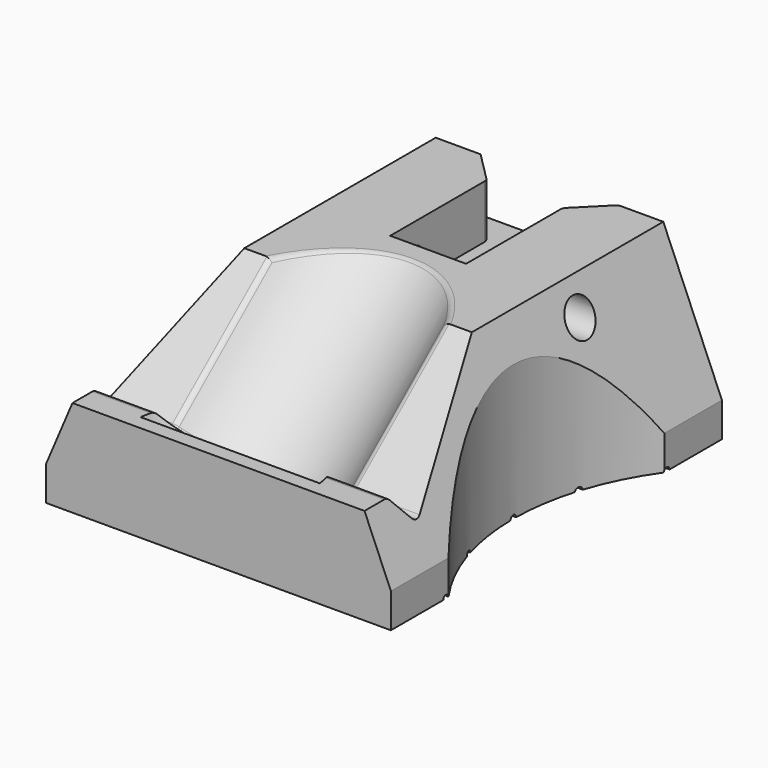
from build123d import *

# Parameters (mm, degrees)
F1_DEPTH  = 120
F2_R      = 2.65
F3_DEPTH  = 50
F4_DEPTH  = 11
F6_R      = 5
F6_R_2    = 2.65
F7_DEPTH  = 25
F10_DEPTH = 25
F11_W     = 11
F11_H     = 9
F12_DEPTH = 15.4995888315
F14_DEPTH = 100.001
F15_R     = 32.5
F16_DEPTH = 100
F17_R     = 27
F18_DEPTH = 3
F19_R     = 1
F20_DEPTH = 100.001
F21_R     = 67.5
F22_DEPTH = 50.001
F23_R     = 2


with BuildPart() as f1:
    # F0 (on Front) → F1 (new body)
    with BuildSketch(Plane.XZ):
        Polygon((-50, 0), (0, 0), (0, 50), (-33, 50), (-50, 10), align=None)
        Polygon((0, 50), (0, 0), (50, 0), (50, 10), (33, 50), align=None)
    extrude(amount=F1_DEPTH)

    # F2 (on Right) → F3 (cut, symmetric)
    with BuildSketch(Plane.YZ):
        with Locations((-35, 41.0004111685)):
            Circle(F2_R)
    extrude(amount=F3_DEPTH, both=True, mode=Mode.SUBTRACT)

    # F2 (on Right) → F4 (cut, symmetric)
    with BuildSketch(Plane.YZ):
        with BuildLine():
            Line((-22.5925706327, 34.5004111685), (0, 34.5004111685))
            Line((0, 34.5004111685), (0, 47.5004111685))
            Line((0, 47.5004111685), (-28.775050201, 47.5004111685))
            ThreePointArc((-28.775050201, 47.5004111685), (-26.7227858494, 44.5342088289), (-26, 41.0004111685))
            ThreePointArc((-26, 41.0004111685), (-26.7227858494, 37.4666135082), (-28.775050201, 34.5004111685))
            Line((-28.775050201, 34.5004111685), (-22.5925706327, 34.5004111685))
        make_face()
        with BuildLine():
            Line((-33.0777759178, 32.2080818652), (-22.5925706327, 34.5004111685))
            Line((-22.5925706327, 34.5004111685), (-28.775050201, 34.5004111685))
            ThreePointArc((-28.775050201, 34.5004111685), (-30.7682386679, 33.0573515547), (-33.0777759178, 32.2080818652))
        make_face()
        with BuildLine():
            Line((-28.775050201, 47.5004111685), (0, 47.5004111685))
            Line((0, 47.5004111685), (0, 56.6271956305))
            Line((0, 56.6271956305), (-27.1273270008, 51.5032727532))
            Line((-27.1273270008, 51.5032727532), (-35.0860282779, 50))
            ThreePointArc((-35.0860282779, 50), (-31.6858522299, 49.3679929314), (-28.775050201, 47.5004111685))
        make_face()
        with BuildLine():
            ThreePointArc((-33.0777759178, 32.2080818652), (-30.7682386679, 33.0573515547), (-28.775050201, 34.5004111685))
            ThreePointArc((-28.775050201, 34.5004111685), (-26.7227858494, 37.4666135082), (-26, 41.0004111685))
            ThreePointArc((-26, 41.0004111685), (-26.7227858494, 44.5342088289), (-28.775050201, 47.5004111685))
            ThreePointArc((-28.775050201, 47.5004111685), (-31.6858522299, 49.3679929314), (-35.0860282779, 50))
            ThreePointArc((-35.0860282779, 50), (-41.394304282, 47.3338835771), (-44, 41.0004111685))
            ThreePointArc((-44, 41.0004111685), (-40.6435796823, 33.9897044731), (-33.0777759178, 32.2080818652))
        make_face()
        with Locations((-35, 41.0004111685)):
            Circle(F2_R, mode=Mode.SUBTRACT)
        with BuildLine():
            Line((-44, 53.045399487), (-44, 41.0004111685))
            ThreePointArc((-44, 41.0004111685), (-41.394304282, 47.3338835771), (-35.0860282779, 50))
            Line((-35.0860282779, 50), (-27.1273270008, 51.5032727532))
            Line((-27.1273270008, 51.5032727532), (-44, 53.045399487))
        make_face()
    extrude(amount=F4_DEPTH, both=True, mode=Mode.SUBTRACT)

    # F6 (on offset) → F7 (cut)
    with BuildSketch(Plane.YZ.offset(24)):
        with Locations((-35, 41.0004111685)):
            Circle(F6_R)
        with Locations((-35, 41.0004111685)):
            Circle(F6_R_2, mode=Mode.SUBTRACT)
    extrude(amount=F7_DEPTH, mode=Mode.SUBTRACT)

    # F9 (on offset) → F10 (cut)
    with BuildSketch(Plane.YZ.offset(-30)):
        Polygon((-39.7920072343, 41.0004111685), (-37.3960036171, 36.8504111685), (-32.6039963829, 36.8504111685), (-30.2079927657, 41.0004111685), (-32.6039963829, 45.1504111685), (-37.3960036171, 45.1504111685), align=None)
    extrude(amount=-F10_DEPTH, mode=Mode.SUBTRACT)

    # F11 (on face) → F12 (cut, through all)
    with BuildSketch(Plane.XY.offset(50)):
        Polygon((-20, 0), (-11, -9), (-11, 0), align=None)
        Polygon((11, 0), (11, -9), (20, 0), align=None)
        with Locations((-5.5, -4.5)):
            Rectangle(F11_W, F11_H)
        with Locations((5.5, -4.5)):
            Rectangle(F11_W, F11_H)
    extrude(amount=-F12_DEPTH, mode=Mode.SUBTRACT)

    # F13 (on face) → F14 (cut, through all)
    with BuildSketch(Plane.YZ.offset(50)):
        Polygon((-105.143306435, 20), (-33.7286775579, 79.9239887514), (-151.3096454964, 75.0189004333), (-120, 37.7055179301), (-111.8561034844, 28), align=None)
        Polygon((-120, 28), (-111.8561034844, 28), (-120, 37.7055179301), align=None)
    extrude(amount=-F14_DEPTH, mode=Mode.SUBTRACT)

    # F15 (on face) → F16 (cut)
    with BuildSketch(Plane(origin=(0, -51.8525474655, -43.5094534539), x_dir=(-1, 0, 0), z_dir=(0, 0.7660444431, 0.6427876097))):
        with Locations((0, 103.0848769822)):
            Circle(F15_R)
    extrude(amount=F16_DEPTH, mode=Mode.SUBTRACT)

    # F17 (on face) → F18 (cut)
    with BuildSketch(Plane(origin=(0, -51.8525474655, -43.5094534539), x_dir=(-1, 0, 0), z_dir=(0, 0.7660444431, 0.6427876097))):
        with Locations((0, 103.0848769822)):
            Circle(F17_R)
    extrude(amount=-F18_DEPTH, mode=Mode.SUBTRACT)

    # F19 (on face) → F20 (cut, through all)
    with BuildSketch(Plane.YZ.offset(50)):
        with Locations((-20, 0)):
            Circle(F19_R)
        with Locations((-40, 0)):
            Circle(F19_R)
        with Locations((-60, 0)):
            Circle(F19_R)
        with Locations((-80, 0)):
            Circle(F19_R)
        with Locations((-100, 0)):
            Circle(F19_R)
    extrude(amount=-F20_DEPTH, mode=Mode.SUBTRACT)

    # F21 (on Top) → F22 (cut, through all)
    with BuildSketch(Plane.XY):
        with Locations((105, -60)):
            Circle(F21_R)
        with Locations((-105, -60)):
            Circle(F21_R)
    extrude(amount=F22_DEPTH, mode=Mode.SUBTRACT)

    # F23
    f23_edges = [f1.edges().sort_by_distance(p)[0] for p in [
        (20, 0, 42.250206),
        (11, -9, 42.250206),
        (-11, -9, 42.250206),
        (-25.476479, -87.267003, 35),
        (25.476479, -87.267003, 35),
        (0, -50.222895, 50),
        (-33.766783, -111.856103, 28),
        (33.766783, -111.856103, 28),
        (-35.613239, -105.143306, 20),
        (35.613239, -105.143306, 20),
        (0, -97.223632, 10.561699),
    ]]
    fillet(f23_edges, radius=F23_R)


solid = f1.part
